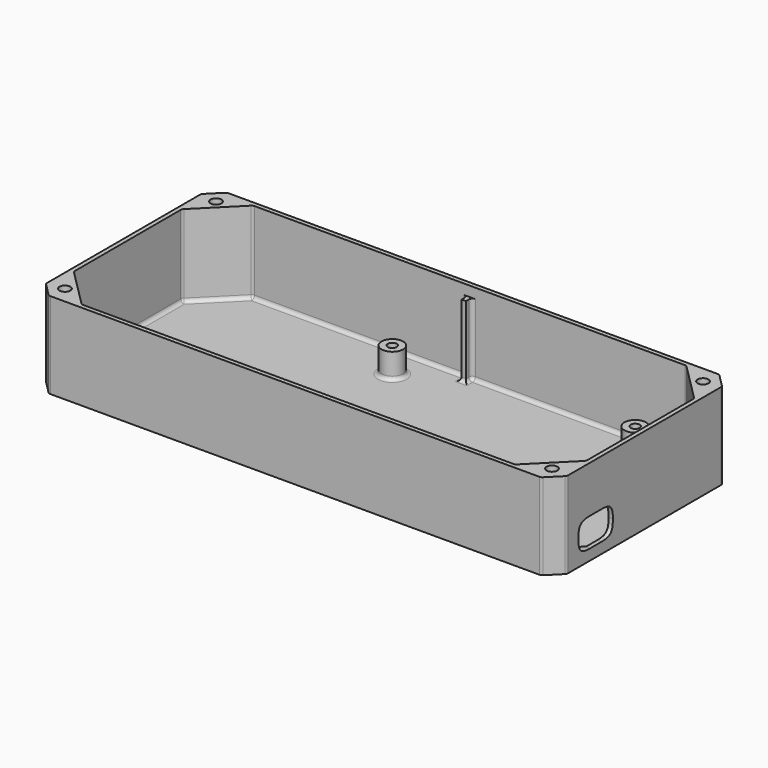
from build123d import *

# Parameters (mm, degrees)
F0_W          = 145
F0_H          = 62
F1_DEPTH      = 24
F2_T          = -1.2
F3_SIZE       = 11
F4_SIZE       = 4
F5_R          = 1.5
F6_DEPTH      = 15
F7_R          = 3
F7_R_2        = 1.25
F8_DEPTH      = 7
F7_W          = 1.2
F7_H          = 2
F9_DEPTH      = 20
F10_W         = 12
F10_H         = 8
F11_DEPTH     = 5.401
F12_T1_DEPTH  = 1.2
F12_T6_DEPTH  = 15.4
F12_T11_DEPTH = 15.4
F13_R         = 1


# Not quite as in the source:
# - a fillet or chamfer that OpenCascade refuses, or shapes differently, is made with other operations: its cross-section is extruded or revolved along the edge and cut away or added
# - a feature names something its author has since deleted; it is built from what else it names


with BuildPart() as f1:
    # F0 (on Top) → F1 (new body)
    with BuildSketch(Plane.XY):
        Rectangle(F0_W, F0_H)
    extrude(amount=F1_DEPTH)

    # F2
    f2_openings = [f1.faces().sort_by_distance(p)[0] for p in [
        (0, 0, 24),
    ]]
    offset(amount=F2_T, openings=f2_openings)

    # F3
    f3_edges = [f1.edges().sort_by_distance(p)[0] for p in [
        (71.3, 29.8, 12.6),
        (-71.3, 29.8, 12.6),
        (-71.3, -29.8, 12.6),
        (71.3, -29.8, 12.6),
    ]]
    chamfer(f3_edges, length=F3_SIZE)

    # F4
    f4_edges = [f1.edges().sort_by_distance(p)[0] for p in [
        (-72.5, -31, 12),
        (-72.5, 31, 12),
        (72.5, -31, 12),
        (72.5, 31, 12),
    ]]
    chamfer(f4_edges, length=F4_SIZE)

    # F5 (on face) → F6 (cut)
    with BuildSketch(Plane.XY.offset(24)):
        with Locations((-67.7798989873, 26.2798989873)):
            Circle(F5_R)
        with Locations((-67.7798989873, -26.2798989873)):
            Circle(F5_R)
        with Locations((67.7798989873, -26.2798989873)):
            Circle(F5_R)
        with Locations((67.7798989873, 26.2798989873)):
            Circle(F5_R)
    extrude(amount=-F6_DEPTH, mode=Mode.SUBTRACT)

    # F7 (on face) → F8 (join)
    with BuildSketch(Plane.XY.offset(1.2)):
        with Locations((-14.5, -21.01)):
            Circle(F7_R)
        with Locations((-14.5, -21.01)):
            Circle(F7_R_2, mode=Mode.SUBTRACT)
        with Locations((50.5, -24.25)):
            Circle(F7_R)
        with Locations((50.5, -24.25)):
            Circle(F7_R_2, mode=Mode.SUBTRACT)
        with Locations((50.5, 24.25)):
            Circle(F7_R)
        with Locations((50.5, 24.25)):
            Circle(F7_R_2, mode=Mode.SUBTRACT)
        with Locations((-14.5, 21.01)):
            Circle(F7_R)
        with Locations((-14.5, 21.01)):
            Circle(F7_R_2, mode=Mode.SUBTRACT)
    extrude(amount=F8_DEPTH)

    # F7 (on face) → F9 (join)
    with BuildSketch(Plane.XY.offset(1.2)):
        with Locations((-0.03283014, 28.8)):
            Rectangle(F7_W, F7_H)
        with Locations((-0.03283014, -28.8)):
            Rectangle(F7_W, F7_H)
    extrude(amount=F9_DEPTH)

    # F10 (on face) → F11 (cut, through all)
    with BuildSketch(Plane.YZ.offset(72.5)):
        with Locations((-17, 7)):
            Rectangle(F10_W, F10_H)
    extrude(amount=-F11_DEPTH, mode=Mode.SUBTRACT)

    # F12: fillet of radius 4 on 4 edges, made by hand

    # F12_s2 → F12_t1 (join)
    with BuildSketch(Plane.YZ.offset(71.3)):
        with BuildLine():
            add(Edge.make_bspline(
                [(-11, 7), (-11, 3), (-15, 3)],
                knots=[0, 0, 0, 1, 1, 1], degree=2, weights=[1, 1.5, 1]))
            Line((-15, 3), (-11, 3))
            Line((-11, 3), (-11, 7))
        make_face()
        with BuildLine():
            add(Edge.make_bspline(
                [(-15, 11), (-11, 11), (-11, 7)],
                knots=[0, 0, 0, 1, 1, 1], degree=2, weights=[1, 1.5, 1]))
            Line((-11, 7), (-11, 11))
            Line((-11, 11), (-15, 11))
        make_face()
    extrude(amount=F12_T1_DEPTH)


with BuildPart() as f12_tool4:
    # F12_s5 → F12_t6 (new body)
    with BuildSketch(Plane.YZ.offset(72.5)):
        with BuildLine():
            add(Edge.make_bspline(
                [(-19, 3), (-23, 3), (-23, 7)],
                knots=[0, 0, 0, 1, 1, 1], degree=2, weights=[1, 1.5, 1]))
            Line((-23, 7), (-23, 3))
            Line((-23, 3), (-19, 3))
        make_face()
    extrude(amount=-F12_T6_DEPTH)

    split(bisect_by=Plane(origin=(45.05, -45.05, 0), x_dir=(0, 0, 1), z_dir=(0.7071067812, -0.7071067812, 0)), keep=Keep.TOP)


with BuildPart() as f1_1:
    add(f1.part)

    # F12_t3: union F12_tool4
    add(f12_tool4.part)


with BuildPart() as f12_tool9:
    # F12_s10 → F12_t11 (new body)
    with BuildSketch(Plane.YZ.offset(72.5)):
        with BuildLine():
            add(Edge.make_bspline(
                [(-19, 11), (-23, 11), (-23, 7)],
                knots=[0, 0, 0, 1, 1, 1], degree=2, weights=[1, 1.5, 1]))
            Line((-23, 7), (-23, 11))
            Line((-23, 11), (-19, 11))
        make_face()
    extrude(amount=-F12_T11_DEPTH)

    split(bisect_by=Plane(origin=(45.05, -45.05, 0), x_dir=(0, 0, 1), z_dir=(0.7071067812, -0.7071067812, 0)), keep=Keep.TOP)


with BuildPart() as f1_2:
    add(f1_1.part)

    # F12_t8: union F12_tool9
    add(f12_tool9.part)

    # F13
    f13_edges = [f1_2.edges().sort_by_distance(p)[0] for p in [
        (-60.3, 29.8, 12.6),
        (-71.3, 18.8, 12.6),
        (60.3, 29.8, 12.6),
        (71.3, 18.8, 12.6),
        (60.3, -29.8, 12.6),
        (-60.3, -29.8, 12.6),
        (-71.3, -18.8, 12.6),
        (-72.5, -27, 12),
        (-68.5, -31, 12),
        (68.5, -31, 12),
        (72.5, -27, 12),
        (72.5, 27, 12),
        (68.5, 31, 12),
        (-68.5, 31, 12),
        (-72.5, 27, 12),
        (71.3, -18.8, 2.1),
        (71.3, -18.8, 17.5),
        (71.3, 0, 1.2),
        (65.8, 24.3, 1.2),
        (30.433585, 29.8, 1.2),
        (-30.466415, 29.8, 1.2),
        (-65.8, 24.3, 1.2),
        (-71.3, 0, 1.2),
        (-17.5, 21.01, 1.2),
        (47.5, 24.25, 1.2),
        (-17.5, -21.01, 1.2),
        (-65.8, -24.3, 1.2),
        (-30.466415, -29.8, 1.2),
        (30.433585, -29.8, 1.2),
        (47.5, -24.25, 1.2),
        (65.8, -24.3, 1.2),
        (-0.63283, -29.8, 11.2),
        (0.56717, -29.8, 11.2),
        (0.56717, 29.8, 11.2),
        (-0.63283, 29.8, 11.2),
        (-0.63283, 28.8, 1.2),
        (-0.03283, 27.8, 1.2),
        (0.56717, 28.8, 1.2),
        (-0.03283, -27.8, 1.2),
        (-0.63283, -28.8, 1.2),
        (0.56717, -28.8, 1.2),
    ]]
    fillet(f13_edges, radius=F13_R)


solid = f1_2.part
